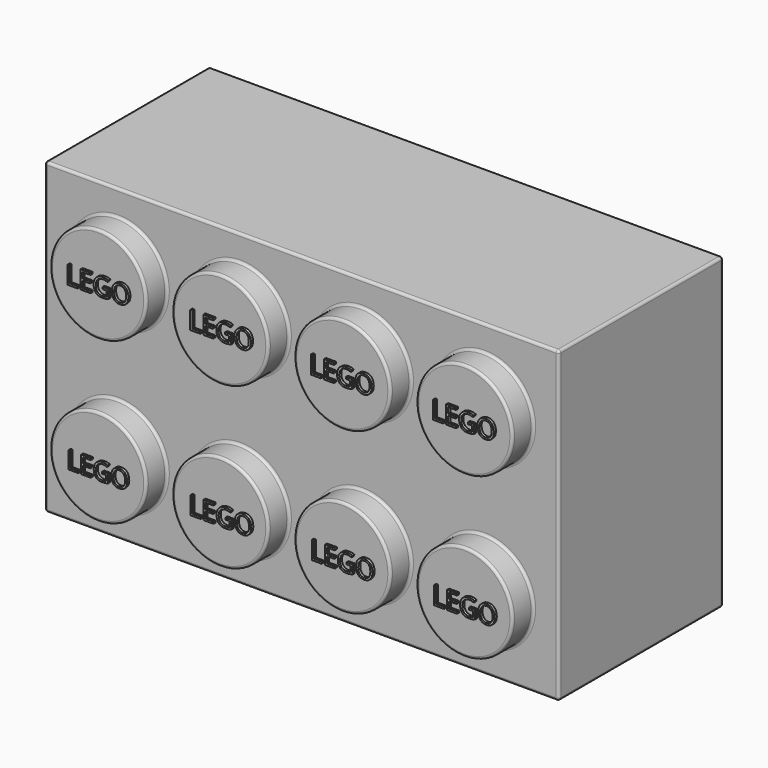
from build123d import *

# Parameters (mm, degrees)
F0_W           = 50.8
F0_H           = 30.48
F1_DEPTH       = 20.32
F2_T           = -2.54
F3_R           = 4.7625
F4_DEPTH       = 2.54
F5_R           = 0.254
F6_TEXT_SIZE   = 2.4786601744
F6_TEXT_SIZE_2 = 2.4768769638
F6_TEXT_SIZE_3 = 2.3895360725
F7_DEPTH       = 0.254


# Not quite as in the source:
# - Text() gives the source's letters only with a copy of the font that has no kerning and outlines rounded to 1/6400 em; it was checked with that copy


with BuildPart() as f1:
    # F0 (on Front) → F1 (new body)
    with BuildSketch(Plane.XZ):
        with Locations((4.3208375573, -2.8363485902)):
            Rectangle(F0_W, F0_H)
    extrude(amount=F1_DEPTH)

    # F2
    f2_openings = [f1.faces().sort_by_distance(p)[0] for p in [
        (4.320838, 0, -2.836349),
    ]]
    offset(amount=F2_T, openings=f2_openings)

    # F3 (on face) → F4 (join)
    with BuildSketch(Plane.XZ.offset(20.32)):
        with Locations((22.4183375573, -10.7738485902)):
            Circle(F3_R)
        with Locations((22.4183375573, 5.1011514098)):
            Circle(F3_R)
        with Locations((10.3533375573, 5.1011514098)):
            Circle(F3_R)
        with Locations((10.3533375573, -10.7738485902)):
            Circle(F3_R)
        with Locations((-13.7766624427, 5.1011514098)):
            Circle(F3_R)
        with Locations((-1.7116624427, 5.1011514098)):
            Circle(F3_R)
        with Locations((-1.7116624427, -10.7738485902)):
            Circle(F3_R)
        with Locations((-13.7766624427, -10.7738485902)):
            Circle(F3_R)
    extrude(amount=F4_DEPTH)

    # F5
    f5_edges = [f1.edges().sort_by_distance(p)[0] for p in [
        (-6.474162, -22.86, -10.773849),
        (5.590838, -22.86, -10.773849),
        (17.655838, -22.86, -10.773849),
        (17.655838, -22.86, 5.101151),
        (5.590838, -22.86, 5.101151),
        (17.655838, -20.32, -10.773849),
        (17.655838, -20.32, 5.101151),
        (5.590838, -20.32, -10.773849),
        (5.590838, -20.32, 5.101151),
        (-6.474162, -20.32, -10.773849),
        (-18.539162, -20.32, -10.773849),
        (-18.539162, -20.32, 5.101151),
        (-6.474162, -20.32, 5.101151),
        (-6.474162, -22.86, 5.101151),
        (-18.539162, -22.86, 5.101151),
        (-18.539162, -22.86, -10.773849),
        (4.320838, -20.32, -18.076349),
        (-21.079162, -10.16, 12.403651),
        (-21.079162, -10.16, -18.076349),
        (-21.079162, 0, -2.836349),
        (-21.079162, -20.32, -2.836349),
        (29.720838, -10.16, -18.076349),
        (29.720838, -10.16, 12.403651),
        (29.720838, 0, -2.836349),
        (29.720838, -20.32, -2.836349),
        (4.320838, 0, 12.403651),
        (4.320838, -20.32, 12.403651),
        (4.320838, 0, -18.076349),
        (4.320838, 0, 9.863651),
        (27.180838, 0, -2.836349),
        (4.320838, 0, -15.536349),
        (-18.539162, 0, -2.836349),
        (27.180838, -8.89, 9.863651),
        (27.180838, -17.78, -2.836349),
        (4.320838, -17.78, -15.536349),
        (4.320838, -17.78, 9.863651),
        (-18.539162, -17.78, -2.836349),
        (-18.539162, -8.89, 9.863651),
        (-18.539162, -8.89, -15.536349),
        (27.180838, -8.89, -15.536349),
    ]]
    fillet(f5_edges, radius=F5_R)

    # F6 (on face) → F7 (join)
    with BuildSketch(Plane.XZ.offset(22.86)):
        with Locations((-16.8307894155, 4.261320839)):
            Text('LEGO', F6_TEXT_SIZE, font='Open Sans', text_align=(TextAlign.LEFT, TextAlign.BOTTOM))
        with Locations((-4.7076388728, 4.2626047507)):
            Text('LEGO', F6_TEXT_SIZE_2, font='Open Sans', text_align=(TextAlign.LEFT, TextAlign.BOTTOM))
        with Locations((7.2255902924, 4.2626047507)):
            Text('LEGO', F6_TEXT_SIZE_2, font='Open Sans', text_align=(TextAlign.LEFT, TextAlign.BOTTOM))
        with Locations((19.2941376008, 4.2626047507)):
            Text('LEGO', F6_TEXT_SIZE_2, font='Open Sans', text_align=(TextAlign.LEFT, TextAlign.BOTTOM))
        with Locations((-16.7184512703, -11.7819812346)):
            Text('LEGO', F6_TEXT_SIZE_3, font='Open Sans', text_align=(TextAlign.LEFT, TextAlign.BOTTOM))
        with Locations((-4.6809539199, -11.8448666763)):
            Text('LEGO', F6_TEXT_SIZE_2, font='Open Sans', text_align=(TextAlign.LEFT, TextAlign.BOTTOM))
        with Locations((7.3022320867, -11.8448666763)):
            Text('LEGO', F6_TEXT_SIZE_2, font='Open Sans', text_align=(TextAlign.LEFT, TextAlign.BOTTOM))
        with Locations((19.3844151217, -11.8448666763)):
            Text('LEGO', F6_TEXT_SIZE_2, font='Open Sans', text_align=(TextAlign.LEFT, TextAlign.BOTTOM))
    extrude(amount=F7_DEPTH)


solid = f1.part
